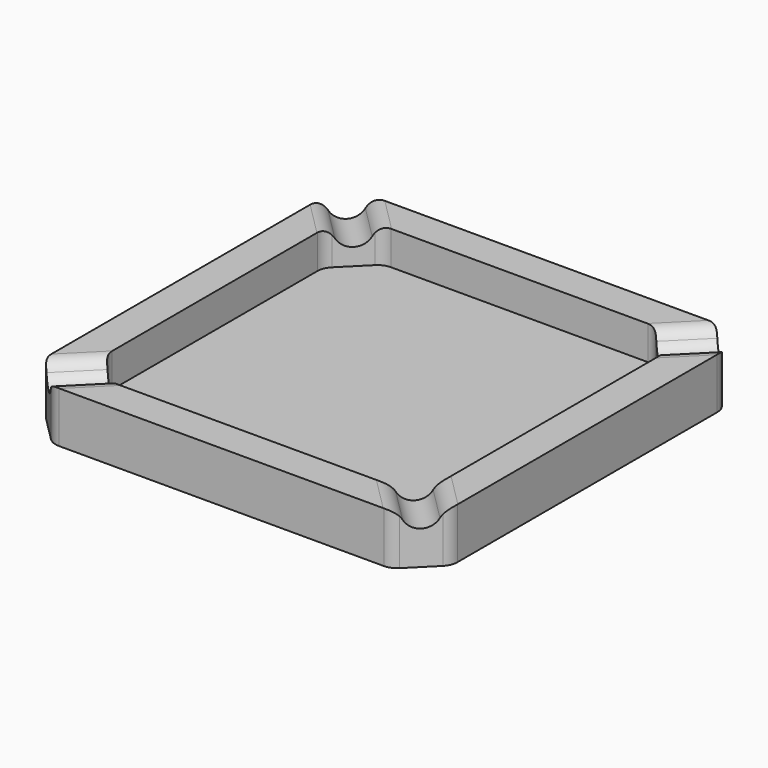
from build123d import *

# Parameters (mm, degrees)
F1_DEPTH      = 15
F3_DEPTH      = 10
F5_R          = 5
F6_DEPTH      = 15
F8_R          = 5
F9_DEPTH      = 15
F11_R         = 5
F12_DEPTH     = 15
F14_R         = 5
F15_DEPTH     = 15
F16_T1_DEPTH  = 32.443405813
F16_T3_DEPTH  = 32.443405813
F16_T5_DEPTH  = 32.443405813
F16_T7_DEPTH  = 32.443405813
F16_T9_DEPTH  = 32.443405813
F16_T11_DEPTH = 32.443405813
F16_T13_DEPTH = 32.443405813
F16_T15_DEPTH = 32.443405813
F17_R         = 5
F18_R         = 5


# Not quite as in the source:
# - a fillet or chamfer that OpenCascade refuses, or shapes differently, is made with other operations: its cross-section is extruded or revolved along the edge and cut away or added


with BuildPart() as f1:
    # F0 (on Top) → F1 (new body)
    with BuildSketch(Plane.XY):
        Polygon((50, 60), (-50, 60), (-60, 50), (-60, -50), (-50, -60), (50, -60), (60, -50), (60, 50), align=None)
    extrude(amount=F1_DEPTH)

    # F2 (on face) → F3 (cut)
    with BuildSketch(Plane.XY.offset(15)):
        Polygon((40, 50), (-40, 50), (-50, 40), (-50, -40), (-40, -50), (40, -50), (50, -40), (50, 40), align=None)
    extrude(amount=-F3_DEPTH, mode=Mode.SUBTRACT)

    # F5 (on offset) → F6 (cut)
    with BuildSketch(Plane(origin=(-55.0707106781, 55.0707106781, 0), x_dir=(-0.7071067812, -0.7071067812, 0), z_dir=(-0.7071067812, 0.7071067812, 0))):
        with Locations((0, 15)):
            Circle(F5_R)
    extrude(amount=-F6_DEPTH, mode=Mode.SUBTRACT)

    # F8 (on offset) → F9 (cut)
    with BuildSketch(Plane(origin=(55.0707106781, 55.0707106781, 0), x_dir=(-0.7071067812, 0.7071067812, 0), z_dir=(0.7071067812, 0.7071067812, 0))):
        with Locations((0, 15)):
            Circle(F8_R)
    extrude(amount=-F9_DEPTH, mode=Mode.SUBTRACT)

    # F11 (on offset) → F12 (cut)
    with BuildSketch(Plane(origin=(55.0707106781, -55.0707106781, 0), x_dir=(0.7071067812, 0.7071067812, 0), z_dir=(0.7071067812, -0.7071067812, 0))):
        with Locations((0, 15)):
            Circle(F11_R)
    extrude(amount=-F12_DEPTH, mode=Mode.SUBTRACT)

    # F14 (on offset) → F15 (cut)
    with BuildSketch(Plane(origin=(-55.0707106781, -55.0707106781, 0), x_dir=(0.7071067812, -0.7071067812, 0), z_dir=(-0.7071067812, -0.7071067812, 0))):
        with Locations((0, 15)):
            Circle(F14_R)
    extrude(amount=-F15_DEPTH, mode=Mode.SUBTRACT)

    # F16: fillet of radius 5 on 8 edges, made by hand

    # F16_s2 → F16_t1 (cut)
    with BuildSketch(Plane(origin=(-61.4704761276, 61.4704761276, 0), x_dir=(0, 0, 1), z_dir=(0.7071067812, -0.7071067812, 0))):
        with BuildLine():
            ThreePointArc((15, 8.6602540378), (14.3301270189, 6.1602540378), (12.5, 4.3301270189))
            ThreePointArc((12.5, 4.3301270189), (13.7059047745, 4.8296291314), (15, 5))
            Line((15, 5), (15, 8.6602540378))
        make_face()
    extrude(amount=F16_T1_DEPTH, mode=Mode.SUBTRACT)

    # F16_s4 → F16_t3 (cut)
    with BuildSketch(Plane(origin=(-38.5295238724, 38.5295238724, 0), x_dir=(0, 0, 1), z_dir=(-0.7071067812, 0.7071067812, 0))):
        with BuildLine():
            ThreePointArc((15, 8.6602540378), (14.3301270189, 6.1602540378), (12.5, 4.3301270189))
            ThreePointArc((12.5, 4.3301270189), (13.7059047745, 4.8296291314), (15, 5))
            Line((15, 5), (15, 8.6602540378))
        make_face()
    extrude(amount=F16_T3_DEPTH, mode=Mode.SUBTRACT)

    # F16_s6 → F16_t5 (cut)
    with BuildSketch(Plane(origin=(-38.5295238724, -38.5295238724, 0), x_dir=(0, 0, 1), z_dir=(-0.7071067812, -0.7071067812, 0))):
        with BuildLine():
            ThreePointArc((15, 8.6602540378), (14.3301270189, 6.1602540378), (12.5, 4.3301270189))
            ThreePointArc((12.5, 4.3301270189), (13.7059047745, 4.8296291314), (15, 5))
            Line((15, 5), (15, 8.6602540378))
        make_face()
    extrude(amount=F16_T5_DEPTH, mode=Mode.SUBTRACT)

    # F16_s8 → F16_t7 (cut)
    with BuildSketch(Plane(origin=(-61.4704761276, -61.4704761276, 0), x_dir=(0, 0, 1), z_dir=(0.7071067812, 0.7071067812, 0))):
        with BuildLine():
            ThreePointArc((12.5, 4.3301270189), (14.3301270189, 6.1602540378), (15, 8.6602540378))
            Line((15, 8.6602540378), (15, 5))
            ThreePointArc((15, 5), (13.7059047745, 4.8296291314), (12.5, 4.3301270189))
        make_face()
    extrude(amount=F16_T7_DEPTH, mode=Mode.SUBTRACT)

    # F16_s10 → F16_t9 (cut)
    with BuildSketch(Plane(origin=(61.4704761276, -61.4704761276, 0), x_dir=(0, 0, 1), z_dir=(-0.7071067812, 0.7071067812, 0))):
        with BuildLine():
            ThreePointArc((15, 8.6602540378), (14.3301270189, 6.1602540378), (12.5, 4.3301270189))
            ThreePointArc((12.5, 4.3301270189), (13.7059047745, 4.8296291314), (15, 5))
            Line((15, 5), (15, 8.6602540378))
        make_face()
    extrude(amount=F16_T9_DEPTH, mode=Mode.SUBTRACT)

    # F16_s12 → F16_t11 (cut)
    with BuildSketch(Plane(origin=(38.5295238724, -38.5295238724, 0), x_dir=(0, 0, 1), z_dir=(0.7071067812, -0.7071067812, 0))):
        with BuildLine():
            ThreePointArc((12.5, 4.3301270189), (14.3301270189, 6.1602540378), (15, 8.6602540378))
            Line((15, 8.6602540378), (15, 5))
            ThreePointArc((15, 5), (13.7059047745, 4.8296291314), (12.5, 4.3301270189))
        make_face()
    extrude(amount=F16_T11_DEPTH, mode=Mode.SUBTRACT)

    # F16_s14 → F16_t13 (cut)
    with BuildSketch(Plane(origin=(61.4704761276, 61.4704761276, 0), x_dir=(0, 0, 1), z_dir=(-0.7071067812, -0.7071067812, 0))):
        with BuildLine():
            ThreePointArc((15, 8.6602540378), (14.3301270189, 6.1602540378), (12.5, 4.3301270189))
            ThreePointArc((12.5, 4.3301270189), (13.7059047745, 4.8296291314), (15, 5))
            Line((15, 5), (15, 8.6602540378))
        make_face()
    extrude(amount=F16_T13_DEPTH, mode=Mode.SUBTRACT)

    # F16_s16 → F16_t15 (cut)
    with BuildSketch(Plane(origin=(38.5295238724, 38.5295238724, 0), x_dir=(0, 0, 1), z_dir=(0.7071067812, 0.7071067812, 0))):
        with BuildLine():
            ThreePointArc((12.5, 4.3301270189), (14.3301270189, 6.1602540378), (15, 8.6602540378))
            Line((15, 8.6602540378), (15, 5))
            ThreePointArc((15, 5), (13.7059047745, 4.8296291314), (12.5, 4.3301270189))
        make_face()
    extrude(amount=F16_T15_DEPTH, mode=Mode.SUBTRACT)

    # F17
    f17_edges = [f1.edges().sort_by_distance(p)[0] for p in [
        (-60, 50, 7.370363),
        (-50, 60, 7.370363),
        (-60, -50, 7.370363),
        (-50, -60, 7.370363),
        (50, -60, 7.370363),
        (60, -50, 7.370363),
        (60, 50, 7.370363),
        (50, 60, 7.370363),
    ]]
    fillet(f17_edges, radius=F17_R)

    # F18
    f18_edges = [f1.edges().sort_by_distance(p)[0] for p in [
        (-40, -50, 9.870363),
        (-50, -40, 9.870363),
        (-50, 40, 9.870363),
        (-40, 50, 9.870363),
        (40, 50, 9.870363),
        (50, 40, 9.870363),
        (50, -40, 9.870363),
        (40, -50, 9.870363),
    ]]
    fillet(f18_edges, radius=F18_R)


solid = f1.part
